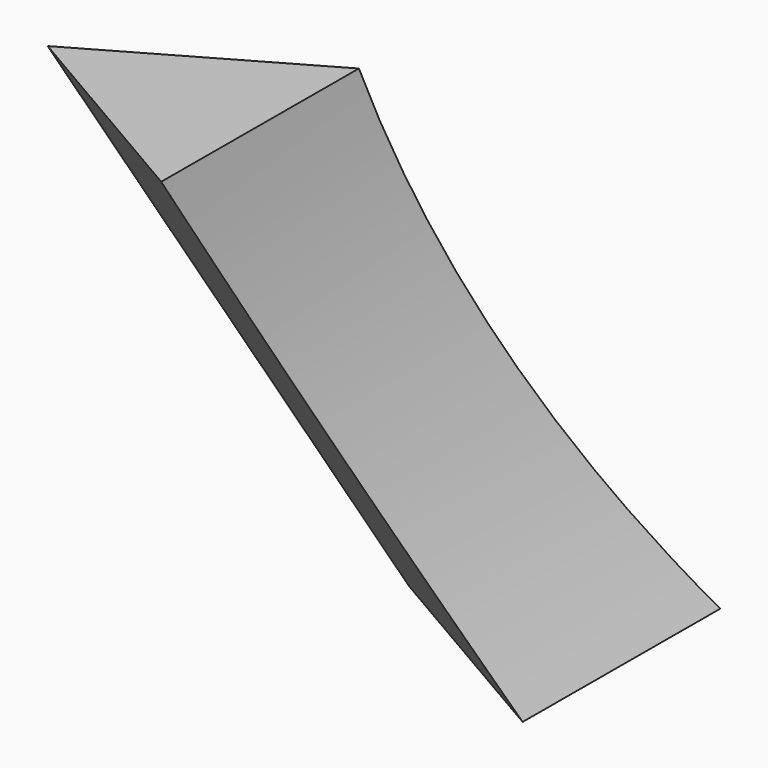
from build123d import *

# Parameters (mm, degrees)
F12_DEPTH = 113.538


# Not quite as in the source:
# - a variable given as a bare number and used for a length is read in inches; the dataset says mm whatever the document's units were


with BuildPart() as f6:
    # F5 (on offset) → F6 section 0
    with BuildSketch(Plane.XY.offset(152.4)):
        Polygon((-40.361484817, -100.3983795552), (-40.0788063243, -24.198903882), (-106.2108272587, -62.0538349628), align=None)
    # F1 (on Top) → F6 section 1
    with BuildSketch(Plane.XY):
        Polygon((21.8555546497, -38.1813400885), (22.1382331424, 38.0181355847), (-43.993787792, 0.1632045038), align=None)
    loft()

    # F11 (on face) → F12 (cut, symmetric)
    with BuildSketch(Plane(origin=(0, 0, 0), x_dir=(-0.9999931191, 0.0037096915, 0), z_dir=(0.0037096915, 0.9999931191, 0))):
        with BuildLine():
            ThreePointArc((-21.9970452561, 0), (16.987540942, 72.9495345165), (39.9887600767, 152.4))
            Line((39.9887600767, 152.4), (-139.3071115017, 152.4))
            Line((-139.3071115017, 152.4), (-139.3071115017, 0))
            Line((-139.3071115017, 0), (-21.9970452561, 0))
        make_face()
    extrude(amount=F12_DEPTH, both=True, mode=Mode.SUBTRACT)


solid = f6.part
